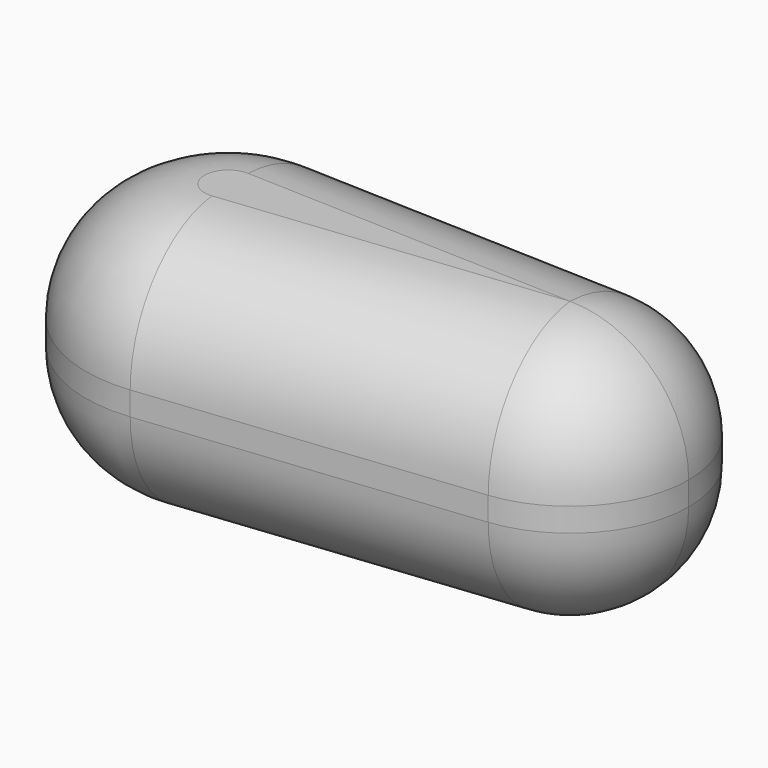
from build123d import *

# Parameters (mm, degrees)
F1_R     = 0.05
F2_DEPTH = 6.6
F3_DEPTH = 0.05
F4_R     = 6


# Not quite as in the source:
# - a feature names something its author has since deleted; it is built from what else it names


with BuildPart() as f2:
    # F1 (on Top) → F2 (new body, symmetric)
    with BuildSketch(Plane.XY):
        with BuildLine():
            ThreePointArc((-22.0188386326, -14.3586602491), (-17.4326418198, -12.0110708593), (-15.5892822956, -7.2))
            ThreePointArc((-15.5892822956, -7.2), (-17.6078830939, -2.2006898163), (-22.5318107159, -0.004605057))
            ThreePointArc((-22.5318107159, -0.004605057), (-29.9846889937, -7.4571428571), (-22.0188386326, -14.3586602491))
        make_face()
        with Locations((-22.7892822956, -7.2)):
            Circle(F1_R, mode=Mode.SUBTRACT)
        with BuildLine():
            ThreePointArc((-22.5318107159, -0.004605057), (-17.6078830939, -2.2006898163), (-15.5892822956, -7.2))
            ThreePointArc((-15.5892822956, -7.2), (-17.4326418198, -12.0110708593), (-22.0188386326, -14.3586602491))
            Line((-22.0188386326, -14.3586602491), (-5.3579636142, -12.5655502076))
            ThreePointArc((-5.3579636142, -12.5655502076), (-11.9961722484, -6.8142857143), (-5.7854403503, -0.6038375475))
            Line((-5.7854403503, -0.6038375475), (-22.5318107159, -0.004605057))
        make_face()
        with BuildLine():
            ThreePointArc((0, -6.6), (-1.682167332, -2.4339081802), (-5.7854403503, -0.6038375475))
            ThreePointArc((-5.7854403503, -0.6038375475), (-11.9961722484, -6.8142857143), (-5.3579636142, -12.5655502076))
            ThreePointArc((-5.3579636142, -12.5655502076), (-1.5361329369, -10.6092257161), (0, -6.6))
        make_face()
        with Locations((-6, -6.6)):
            Circle(F1_R, mode=Mode.SUBTRACT)
        with Locations((-22.7892822956, -7.2)):
            Circle(F1_R)
        with Locations((-6, -6.6)):
            Circle(F1_R)
    extrude(amount=F2_DEPTH, both=True)

    # F1 (on Top) → F3 (cut, symmetric)
    with BuildSketch(Plane.XY):
        with Locations((-22.7892822956, -7.2)):
            Circle(F1_R)
        with Locations((-6, -6.6)):
            Circle(F1_R)
    extrude(amount=F3_DEPTH, both=True, mode=Mode.SUBTRACT)

    # F4
    f4_edges = [f2.edges().sort_by_distance(p)[0] for p in [
        (-29.984689, -7.457143, 6.6),
        (-13.688401, -13.462105, 6.6),
        (-0.003828, -6.385714, 6.6),
        (-14.158626, -0.304221, 6.6),
        (-29.984689, -7.457143, -6.6),
        (-13.688401, -13.462105, -6.6),
        (-0.003828, -6.385714, -6.6),
        (-14.158626, -0.304221, -6.6),
    ]]
    fillet(f4_edges, radius=F4_R)


solid = f2.part
